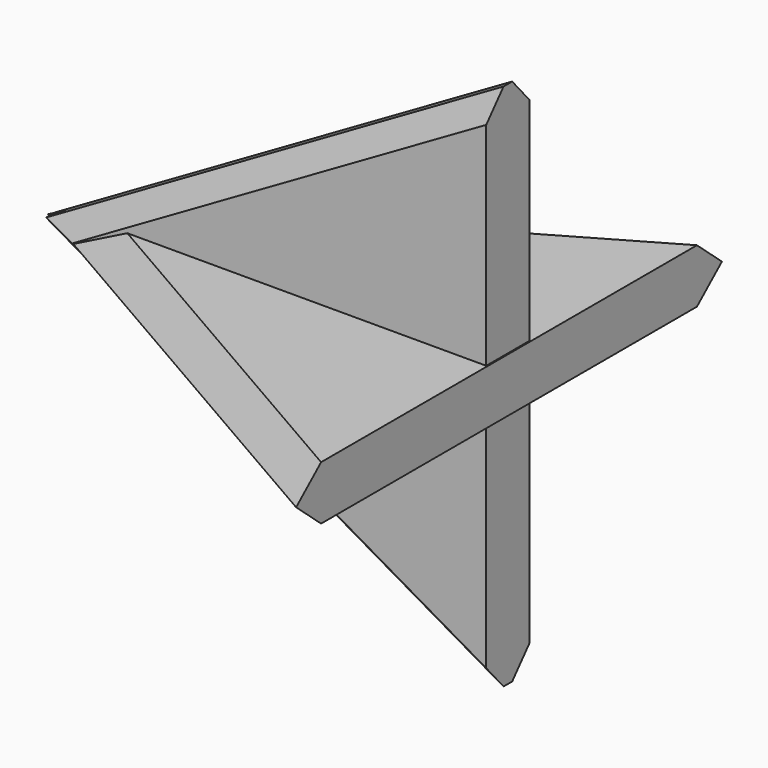
from build123d import *

# Parameters (mm, degrees)
F1_DEPTH = 2.54
F2_SIZE  = 2.53999
F4_DEPTH = 2.54
F5_SIZE  = 2.032


# Not quite as in the source:
# - a fillet or chamfer is up to 0.001 mm smaller than in the source, because OpenCascade refuses the exact size


with BuildPart() as f1:
    # F0 (on Top) → F1 (new body, symmetric)
    with BuildSketch(Plane.XY):
        Polygon((14.4337567297, -25), (14.4337567297, 25), (-28.8675134595, 0), align=None)
    extrude(amount=F1_DEPTH, both=True)

    # F2 (size 2.54 in the source; OpenCascade refuses exactly that, so slightly less here)
    f2_edges = [f1.edges().sort_by_distance(p)[0] for p in [
        (-7.216878, 12.5, 2.54),
        (-7.216878, -12.5, 2.54),
        (-7.216878, -12.5, -2.54),
        (-7.216878, 12.5, -2.54),
    ]]
    chamfer(f2_edges, length=F2_SIZE)

    # F3 (on Front) → F4 (join, symmetric)
    with BuildSketch(Plane.XZ):
        Polygon((14.3245235085, -24.810802511), (14.3245235085, 24.810802511), (-28.6490470171, 0), align=None)
    extrude(amount=F4_DEPTH, both=True)

    # F5
    f5_edges = [f1.edges().sort_by_distance(p)[0] for p in [
        (-7.162262, 2.54, 12.405401),
        (-7.162262, -2.54, 12.405401),
        (-7.162262, -2.54, -12.405401),
        (-7.162262, 2.54, -12.405401),
    ]]
    chamfer(f5_edges, length=F5_SIZE)


solid = f1.part
